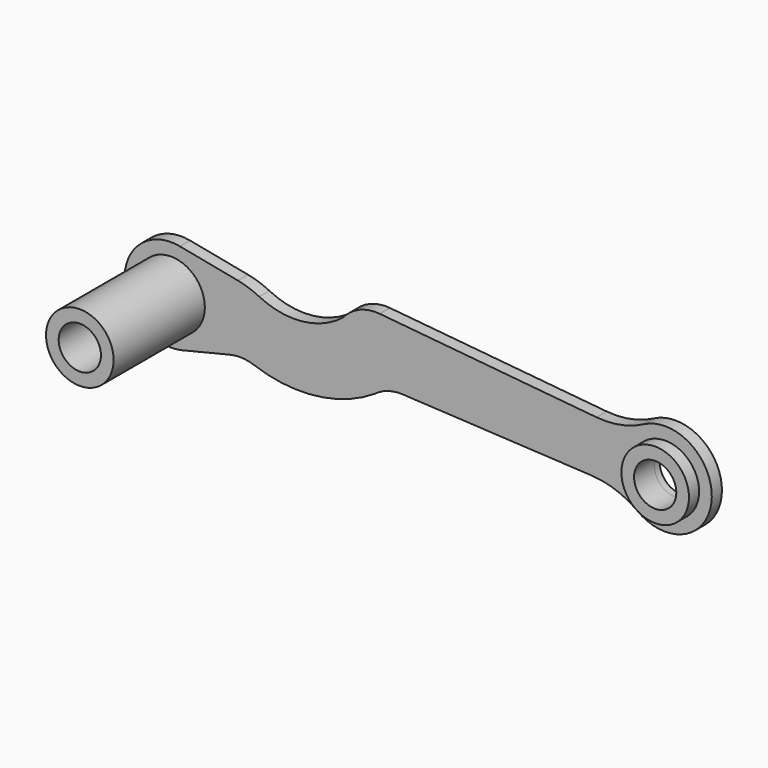
from build123d import *

# Parameters (mm, degrees)
F0_R     = 40
F1_DEPTH = 15
F0_R_2   = 25
F2_DEPTH = 150
F3_DEPTH = 30
F4_DEPTH = 8


# Not quite as in the source:
# - ends of sketch curves that miss each other by under 0.0002 mm in the source are joined


with BuildPart() as f1:
    # F0 (on Front) → F1 (new body)
    with BuildSketch(Plane.XZ):
        with BuildLine():
            ThreePointArc((136.9199448282, 386.2104516544), (124.4705090254, 391.3857217921), (111.4380638613, 394.8393062852))
            Line((111.4380638613, 394.8393062852), (42.918713, 408.129393))
            ThreePointArc((42.918713, 408.129393), (-22.539049679, 352.8547276711), (45.4216669824, 300.6881840726))
            Line((45.4216669824, 300.6881840726), (102.160582, 314.462893))
            ThreePointArc((102.160582, 314.462893), (116.5305641711, 315.8079808018), (130.6860790256, 312.992479072))
            ThreePointArc((130.6860790256, 312.992479072), (204.0553442227, 304.6657026983), (273.5865736459, 329.5211325506))
            ThreePointArc((273.5865736459, 329.5211325506), (289.1363732598, 337.5026610827), (306.4832439925, 339.6444218586))
            Line((306.4832439925, 339.6444218586), (530.552186, 327.792845))
            ThreePointArc((530.552186, 327.792845), (559.0680406559, 322.0478617496), (584.7240709532, 308.3392179368))
            ThreePointArc((584.7240709532, 308.3392179368), (672.2592374085, 348.3136045992), (591.9275499624, 401.2964030718))
            ThreePointArc((591.9275499624, 401.2964030718), (564.8093719906, 391.7707004398), (536.1018479581, 390.3520205594))
            Line((536.1018479581, 390.3520205594), (279.382043, 414.771009))
            ThreePointArc((279.382043, 414.771009), (255.4725507994, 411.172762836), (236.0470033399, 396.7762595435))
            ThreePointArc((236.0470033399, 396.7762595435), (188.0244125036, 377.0364695299), (136.9199448282, 386.2104516544))
        make_face()
        with Locations((32.446032, 354.135662)):
            Circle(F0_R, mode=Mode.SUBTRACT)
        with Locations((617.423637, 352.562949)):
            Circle(F0_R, mode=Mode.SUBTRACT)
    extrude(amount=F1_DEPTH)

    # F0 (on Front) → F2 (join)
    with BuildSketch(Plane.XZ):
        with Locations((32.446032, 354.135662)):
            Circle(F0_R)
        with Locations((32.446032, 354.135662)):
            Circle(F0_R_2, mode=Mode.SUBTRACT)
    extrude(amount=F2_DEPTH)

    # F0 (on Front) → F3 (join)
    with BuildSketch(Plane.XZ):
        with Locations((617.423637, 352.562949)):
            Circle(F0_R)
        with Locations((617.423637, 352.562949)):
            Circle(F0_R_2, mode=Mode.SUBTRACT)
    extrude(amount=F3_DEPTH)

    # F0 (on Front) → F4 (join)
    with BuildSketch(Plane.XZ):
        with Locations((617.423637, 352.562949)):
            Circle(F0_R)
        with Locations((617.423637, 352.562949)):
            Circle(F0_R_2, mode=Mode.SUBTRACT)
    extrude(amount=-F4_DEPTH)


solid = f1.part
